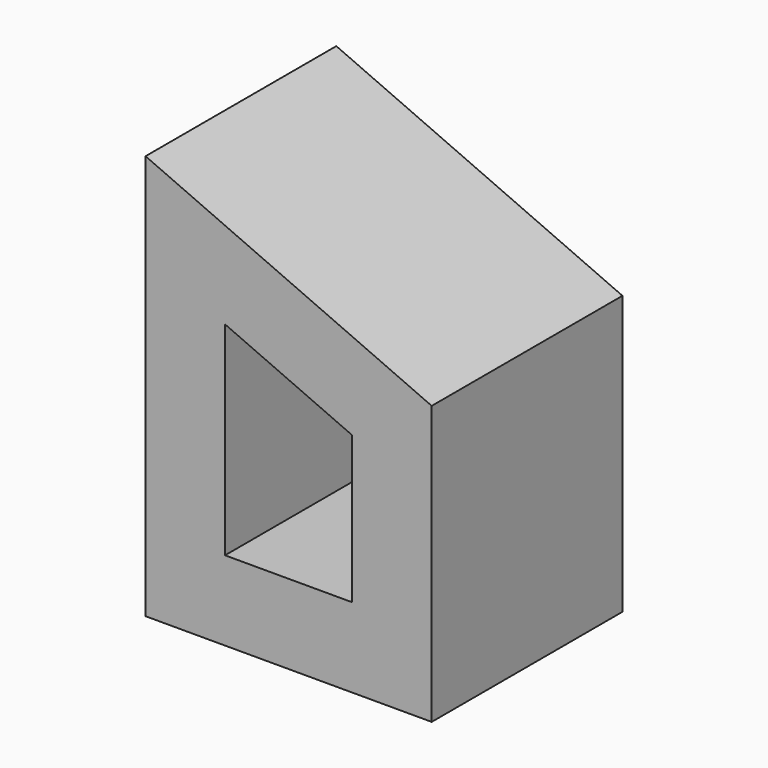
from build123d import *

# Parameters (mm, degrees)
F1_DEPTH = 3000
F2_DEPTH = 250
F4_DEPTH = 140
F5_W     = 1500
F5_H     = 18
F6_DEPTH = 200
F5_W_2   = 400
F5_W_3   = 800
F5_W_4   = 1200
F7_R     = 7
F8_REACH = 4115.4675487723


with BuildPart() as f1:
    # F0 (on Front) → F1 (new body)
    with BuildSketch(Plane.XZ):
        Polygon((2600, -1000), (2600, 2500.7047850388), (-1000, 4095.6675588991), (-1000, -1000), align=None)
        Polygon((1600, 0), (0, 0), (0, 2558.8723439379), (1600, 1850), align=None, mode=Mode.SUBTRACT)
    extrude(amount=F1_DEPTH)

    # F0 (on Front) → F2 (join)
    with BuildSketch(Plane.XZ):
        Polygon((0, 2558.8723439379), (0, 0), (1600, 0), (1600, 1850), align=None)
    extrude(amount=F2_DEPTH)


with BuildPart() as f4:
    # F3 (on face) → F4 (new body)
    with BuildSketch(Plane.XZ.offset(250)):
        Polygon((1400, 750), (200, 750), (200, 150), (1400, 150), (1400, 0), (1450, 0), (1450, 250), (1400, 250), align=None)
    extrude(amount=F4_DEPTH)


with BuildPart() as f6:
    # F5 (on face) → F6 (new body)
    with BuildSketch(Plane.XZ.offset(250)):
        with Locations((800, 859)):
            Rectangle(F5_W, F5_H)
    extrude(amount=F6_DEPTH)


with BuildPart() as f6b:
    # F5 (on face) → F6, piece 2 (new body)
    with BuildSketch(Plane.XZ.offset(250)):
        with Locations((1350, 1227)):
            Rectangle(F5_W_2, F5_H)
    extrude(amount=F6_DEPTH)


with BuildPart() as f6c:
    # F5 (on face) → F6, piece 3 (new body)
    with BuildSketch(Plane.XZ.offset(250)):
        with Locations((450, 1127)):
            Rectangle(F5_W_3, F5_H)
    extrude(amount=F6_DEPTH)


with BuildPart() as f6d:
    # F5 (on face) → F6, piece 4 (new body)
    with BuildSketch(Plane.XZ.offset(250)):
        with Locations((450, 1395)):
            Rectangle(F5_W_3, F5_H)
    extrude(amount=F6_DEPTH)


with BuildPart() as f6e:
    # F5 (on face) → F6, piece 5 (new body)
    with BuildSketch(Plane.XZ.offset(250)):
        with Locations((800, 1613)):
            Rectangle(F5_W, F5_H)
    extrude(amount=F6_DEPTH)


with BuildPart() as f6f:
    # F5 (on face) → F6, piece 6 (new body)
    with BuildSketch(Plane.XZ.offset(250)):
        with Locations((450, 2049)):
            Rectangle(F5_W_3, F5_H)
    extrude(amount=F6_DEPTH)


with BuildPart() as f6g:
    # F5 (on face) → F6, piece 7 (new body)
    with BuildSketch(Plane.XZ.offset(250)):
        with Locations((650, 1831)):
            Rectangle(F5_W_4, F5_H)
    extrude(amount=F6_DEPTH)


with BuildPart() as f8:
    f8_end = f1.part.faces().sort_by_distance((800, -1625, 2204.4361719689))[0]
    # F7 (on face) → F8 (new body, up to a face of F1 that its end follows)
    with BuildSketch(Plane.XY):
        with Locations((100, -275)):
            Circle(F7_R)
    f8_long = extrude(amount=F8_REACH, mode=Mode.PRIVATE)
    add(split(f8_long, bisect_by=f8_end, keep=Keep.TOP, mode=Mode.PRIVATE))


with BuildPart() as f8b:
    f8_2_end = f1.part.faces().sort_by_distance((800, -1625, 2204.4361719689))[0]
    # F7 (on face) → F8, piece 2 (new body, up to a face of F1 that its end follows)
    with BuildSketch(Plane.XY):
        with Locations((100, -425)):
            Circle(F7_R)
    f8_2_long = extrude(amount=F8_REACH, mode=Mode.PRIVATE)
    add(split(f8_2_long, bisect_by=f8_2_end, keep=Keep.TOP, mode=Mode.PRIVATE))


with BuildPart() as f8c:
    f8_3_end = f1.part.faces().sort_by_distance((800, -1625, 2204.4361719689))[0]
    # F7 (on face) → F8, piece 3 (new body, up to a face of F1 that its end follows)
    with BuildSketch(Plane.XY):
        with Locations((1500, -425)):
            Circle(F7_R)
    f8_3_long = extrude(amount=F8_REACH, mode=Mode.PRIVATE)
    add(split(f8_3_long, bisect_by=f8_3_end, keep=Keep.TOP, mode=Mode.PRIVATE))


with BuildPart() as f8d:
    f8_4_end = f1.part.faces().sort_by_distance((800, -1625, 2204.4361719689))[0]
    # F7 (on face) → F8, piece 4 (new body, up to a face of F1 that its end follows)
    with BuildSketch(Plane.XY):
        with Locations((1500, -275)):
            Circle(F7_R)
    f8_4_long = extrude(amount=F8_REACH, mode=Mode.PRIVATE)
    add(split(f8_4_long, bisect_by=f8_4_end, keep=Keep.TOP, mode=Mode.PRIVATE))


with BuildPart() as f8e:
    f8_5_end = f1.part.faces().sort_by_distance((800, -1625, 2204.4361719689))[0]
    # F7 (on face) → F8, piece 5 (new body, up to a face of F1 that its end follows)
    with BuildSketch(Plane.XY):
        with Locations((800, -275)):
            Circle(F7_R)
    f8_5_long = extrude(amount=F8_REACH, mode=Mode.PRIVATE)
    add(split(f8_5_long, bisect_by=f8_5_end, keep=Keep.TOP, mode=Mode.PRIVATE))


with BuildPart() as f8f:
    f8_6_end = f1.part.faces().sort_by_distance((800, -1625, 2204.4361719689))[0]
    # F7 (on face) → F8, piece 6 (new body, up to a face of F1 that its end follows)
    with BuildSketch(Plane.XY):
        with Locations((800, -425)):
            Circle(F7_R)
    f8_6_long = extrude(amount=F8_REACH, mode=Mode.PRIVATE)
    add(split(f8_6_long, bisect_by=f8_6_end, keep=Keep.TOP, mode=Mode.PRIVATE))


with BuildPart() as f8g:
    f8_7_end = f1.part.faces().sort_by_distance((800, -1625, 2204.4361719689))[0]
    # F7 (on face) → F8, piece 7 (new body, up to a face of F1 that its end follows)
    with BuildSketch(Plane.XY):
        with Locations((1200, -275)):
            Circle(F7_R)
    f8_7_long = extrude(amount=F8_REACH, mode=Mode.PRIVATE)
    add(split(f8_7_long, bisect_by=f8_7_end, keep=Keep.TOP, mode=Mode.PRIVATE))


with BuildPart() as f8h:
    f8_8_end = f1.part.faces().sort_by_distance((800, -1625, 2204.4361719689))[0]
    # F7 (on face) → F8, piece 8 (new body, up to a face of F1 that its end follows)
    with BuildSketch(Plane.XY):
        with Locations((1200, -425)):
            Circle(F7_R)
    f8_8_long = extrude(amount=F8_REACH, mode=Mode.PRIVATE)
    add(split(f8_8_long, bisect_by=f8_8_end, keep=Keep.TOP, mode=Mode.PRIVATE))


solid = Compound([f1.part, f4.part, f6.part, f6b.part, f6c.part, f6d.part, f6e.part, f6f.part, f6g.part, f8.part, f8b.part, f8c.part, f8d.part, f8e.part, f8f.part, f8g.part, f8h.part])
